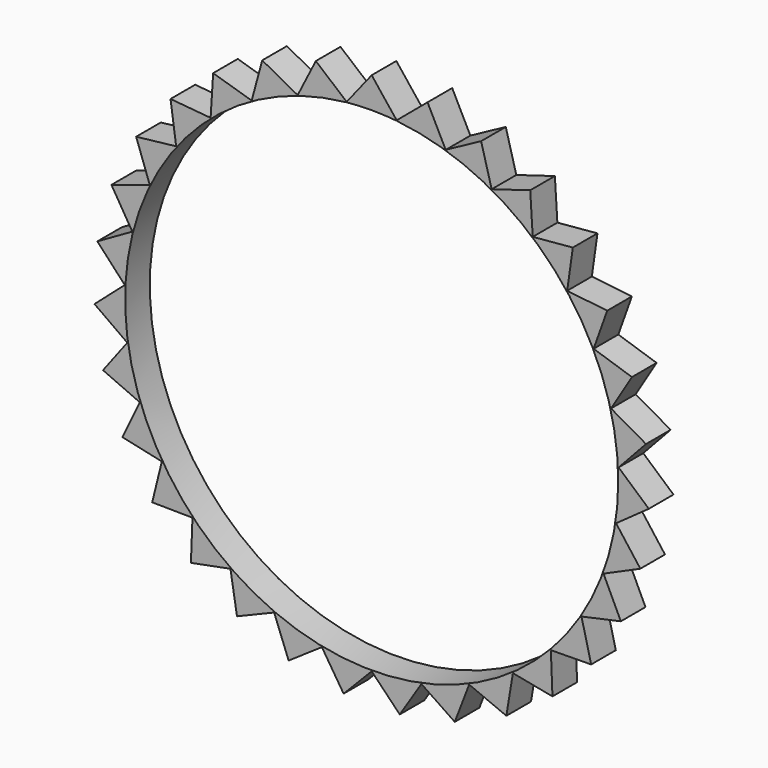
from build123d import *

# Parameters (mm, degrees)
F1_DEPTH = 3.175


# Not quite as in the source:
# - ends of sketch curves that miss each other by under 0.0002 mm in the source are joined


with BuildPart() as f1:
    # F0 (on Front) → F1 (new body)
    with BuildSketch(Plane.XZ):
        with BuildLine():
            ThreePointArc((-2.5175012698, 25.2898644656), (-1.2603037412, 25.3836758526), (0, 25.4149917008))
            Line((0, 25.4149917008), (0, 28.5899917008))
            Line((0, 28.5899917008), (-2.5767820025, 25.3395659531))
            Line((-2.5767820025, 25.3395659531), (-2.5175012698, 25.2898644656))
        make_face()
        with BuildLine():
            Line((0, 28.5899917008), (0, 25.4149917008))
            ThreePointArc((0, 25.4149917008), (1.2603700069, 25.3837316461), (2.5176362485, 25.2899694843))
            Line((2.5176362485, 25.2899694843), (2.5767820025, 25.3395659531))
            Line((2.5767820025, 25.3395659531), (0, 28.5899917008))
        make_face()
    extrude(amount=F1_DEPTH)


with BuildPart() as f1b:
    # F0 (on Front) → F1, piece 2 (new body)
    with BuildSketch(Plane.XZ):
        with BuildLine():
            ThreePointArc((25.400594653, 0.0149917078), (-17.0063726111, -18.850931659), (-2.624843495, 25.2789398262))
            Line((-2.624843495, 25.2789398262), (-2.5767820025, 25.3395659531))
            Line((-2.5767820025, 25.3395659531), (-5.7551230187, 28.0047528911))
            Line((-5.7551230187, 28.0047528911), (-7.6248522496, 24.3021611457))
            Line((-7.6248522496, 24.3021611457), (-11.2746306249, 26.2729962076))
            Line((-11.2746306249, 26.2729962076), (-12.3607601497, 22.2698230056))
            Line((-12.3607601497, 22.2698230056), (-16.3325535285, 23.4656199724))
            Line((-16.3325535285, 23.4656199724), (-16.5906170769, 19.3257556951))
            Line((-16.5906170769, 19.3257556951), (-20.7218197717, 19.6975584985))
            Line((-20.7218197717, 19.6975584985), (-20.1412521917, 15.5904896757))
            Line((-20.1412521917, 15.5904896757), (-24.2627322787, 15.1230766653))
            Line((-24.2627322787, 15.1230766653), (-22.8673020753, 11.2169471773))
            Line((-22.8673020753, 11.2169471773), (-26.8103256755, 9.9294542965))
            Line((-26.8103256755, 9.9294542965), (-24.6571619251, 6.3841815434))
            Line((-24.6571619251, 6.3841815434), (-28.260301189, 4.3293189021))
            Line((-28.260301189, 4.3293189021), (-25.4375546686, 1.290046767))
            Line((-25.4375546686, 1.290046767), (-28.5532966515, -1.4480593168))
            Line((-28.5532966515, -1.4480593168), (-25.1765309352, -3.8569026755))
            Line((-25.1765309352, -3.8569026755), (-27.6773167941, -7.1661538171))
            Line((-27.6773167941, -7.1661538171), (-23.8847770672, -8.8459500694))
            Line((-23.8847770672, -8.8459500694), (-25.6682243353, -12.5908651381))
            Line((-25.6682243353, -12.5908651381), (-21.6151776197, -13.4728432281))
            Line((-21.6151776197, -13.4728432281), (-22.6082717562, -17.500104961))
            Line((-22.6082717562, -17.500104961), (-18.4606502608, -17.548156602))
            Line((-18.4606502608, -17.548156602), (-18.6227338752, -21.6928884307))
            Line((-18.6227338752, -21.6928884307), (-14.5503417112, -20.9050463828))
            Line((-14.5503417112, -20.9050463828), (-13.8747790811, -24.9975624992))
            Line((-13.8747790811, -24.9975624992), (-10.0443404623, -23.4060811085))
            Line((-10.0443404623, -23.4060811085), (-8.5587892013, -27.2788334219))
            Line((-8.5587892013, -27.2788334219), (-5.1271227347, -24.9488681235))
            Line((-5.1271227347, -24.9488681235), (-2.892401486, -28.4433056992))
            Line((-2.892401486, -28.4433056992), (0, -25.4702455461))
            Line((0, -25.4702455461), (2.892401486, -28.4433056992))
            Line((2.892401486, -28.4433056992), (5.1271227347, -24.9488681235))
            Line((5.1271227347, -24.9488681235), (8.5587892013, -27.2788334219))
            Line((8.5587892013, -27.2788334219), (10.0443404623, -23.4060811085))
            Line((10.0443404623, -23.4060811085), (13.8747790811, -24.9975624992))
            Line((13.8747790811, -24.9975624992), (14.5503417112, -20.9050463828))
            Line((14.5503417112, -20.9050463828), (18.6227338752, -21.6928884307))
            Line((18.6227338752, -21.6928884307), (18.4606502608, -17.548156602))
            Line((18.4606502608, -17.548156602), (22.6082717562, -17.500104961))
            Line((22.6082717562, -17.500104961), (21.6151776197, -13.4728432281))
            Line((21.6151776197, -13.4728432281), (25.6682243353, -12.5908651381))
            Line((25.6682243353, -12.5908651381), (23.8847770672, -8.8459500694))
            Line((23.8847770672, -8.8459500694), (27.6773167941, -7.1661538171))
            Line((27.6773167941, -7.1661538171), (25.1765309352, -3.8569026755))
            Line((25.1765309352, -3.8569026755), (28.5532966515, -1.4480593168))
            Line((28.5532966515, -1.4480593168), (25.4375546686, 1.290046767))
            Line((25.4375546686, 1.290046767), (28.260301189, 4.3293189021))
            Line((28.260301189, 4.3293189021), (24.6571619251, 6.3841815434))
            Line((24.6571619251, 6.3841815434), (26.8103256755, 9.9294542965))
            Line((26.8103256755, 9.9294542965), (22.8673020753, 11.2169471773))
            Line((22.8673020753, 11.2169471773), (24.2627322787, 15.1230766653))
            Line((24.2627322787, 15.1230766653), (20.1412521917, 15.5904896757))
            Line((20.1412521917, 15.5904896757), (20.7218197717, 19.6975584985))
            Line((20.7218197717, 19.6975584985), (16.5906170769, 19.3257556951))
            Line((16.5906170769, 19.3257556951), (16.3325535285, 23.4656199724))
            Line((16.3325535285, 23.4656199724), (12.3607601497, 22.2698230056))
            Line((12.3607601497, 22.2698230056), (11.2746306249, 26.2729962076))
            Line((11.2746306249, 26.2729962076), (7.6248522496, 24.3021611457))
            Line((7.6248522496, 24.3021611457), (5.7551230187, 28.0047528911))
            Line((5.7551230187, 28.0047528911), (2.5767820025, 25.3395659531))
            Line((2.5767820025, 25.3395659531), (2.6247367489, 25.2790744788))
            ThreePointArc((2.6247367489, 25.2790744788), (18.8660817821, 17.0224428802), (25.400594653, 0.0149917078))
        make_face()
    extrude(amount=F1_DEPTH)


solid = Compound([f1.part, f1b.part])
